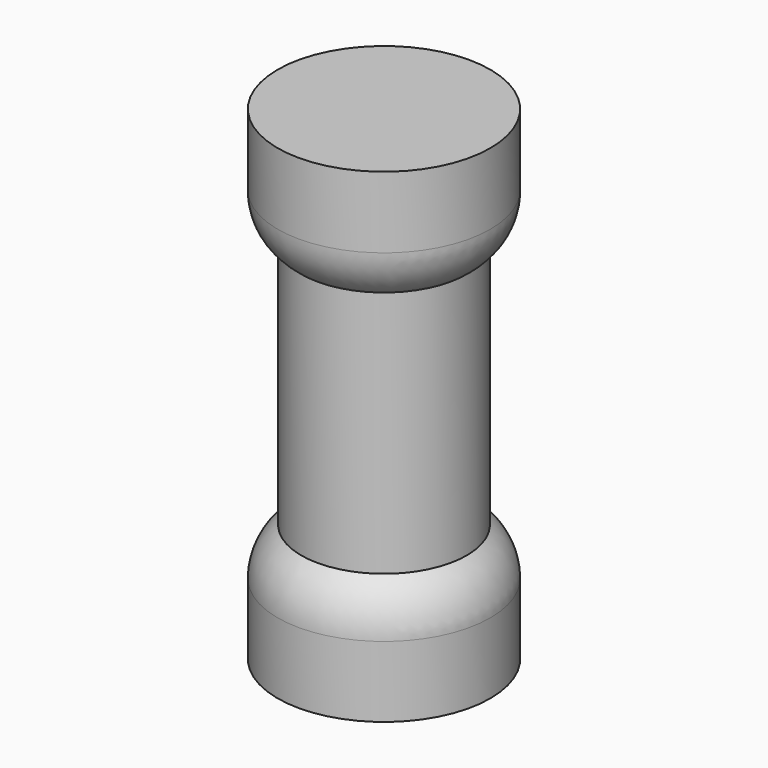
from build123d import *


# Not quite as in the source:
# - a fillet or chamfer that OpenCascade refuses, or shapes differently, is made with other operations: its cross-section is extruded or revolved along the edge and cut away or added


with BuildPart() as f1:
    # F0 (on Right) → F1 (revolve)
    with BuildSketch(Plane.YZ):
        Polygon((-1.8, 0), (0, 0), (0, 8.2), (-1.8, 8.2), (-1.8, 6.2), (-1.4, 6.1908951029), (-1.4, 2), (-1.8, 2), align=None)
    revolve(axis=Axis((0, 0, 4.1), (0, 0, 1)))

    # F2: fillet of radius 1 on 2 edges, made by hand

    # F2_s1 → F2_t2 (revolve, cut)
    with BuildSketch(Plane.YZ):
        with BuildLine():
            ThreePointArc((-1.8, 6.9908951029), (-1.694427191, 6.5436815074), (-1.4, 6.1908951029))
            Line((-1.4, 6.1908951029), (-1.8, 6.2))
            Line((-1.8, 6.2), (-1.8, 6.9908951029))
        make_face()
    revolve(axis=Axis((0, 0, 6.2), (0, 0, 1)), mode=Mode.SUBTRACT)

    # F2_s3 → F2_t4 (revolve, cut)
    with BuildSketch(Plane.YZ):
        with BuildLine():
            ThreePointArc((-1.4, 2), (-1.694427191, 1.6472135955), (-1.8, 1.2))
            Line((-1.8, 1.2), (-1.8, 2))
            Line((-1.8, 2), (-1.4, 2))
        make_face()
    revolve(axis=Axis((0, 0, 2), (0, 0, 1)), mode=Mode.SUBTRACT)


solid = f1.part
